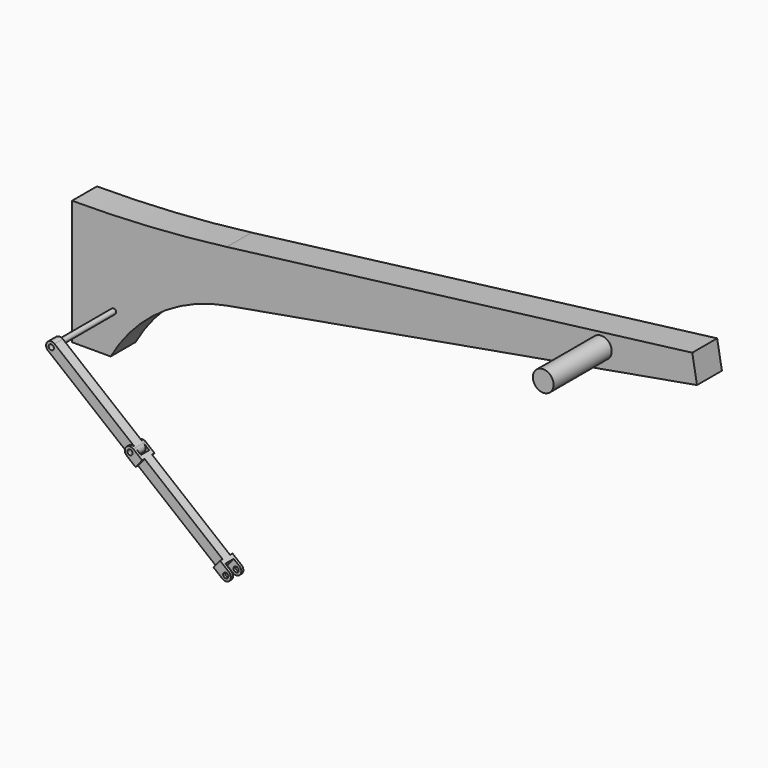
from build123d import *

# Parameters (mm, degrees)
F23_R     = 12.5
F25_DEPTH = 37.5
F24_R     = 12.5
F26_DEPTH = 25
F27_W     = 25
F27_H     = 25
F27_W_2   = 35
F27_W_3   = 482.723958417
F27_H_2   = 15
F28_DEPTH = 594.1776868073
F21_R     = 50
F30_DEPTH = 350
F29_R     = 12.5
F31_R     = 50
F32_DEPTH = 150


# Not quite as in the source:
# - a pattern or mirror of a feature is missing from the dataset's text; its kind, count and spacing are read off the source's solid


with BuildPart() as f25:
    # F23 (on Front) → F25 (new body, symmetric)
    with BuildSketch(Plane.XZ):
        with BuildLine():
            Line((-852.3729289945, 617.7499249904), (-391.0874269249, 245.5438309217))
            ThreePointArc((-391.0874269249, 245.5438309217), (-355.9322933967, 249.3010355502), (-359.6894980253, 284.4561690783))
            Line((-359.6894980253, 284.4561690783), (-820.9750000949, 656.6622631471))
            ThreePointArc((-820.9750000949, 656.6622631471), (-856.130133623, 652.9050585185), (-852.3729289945, 617.7499249904))
        make_face()
        with Locations((-375.3884624751, 265)):
            Circle(F23_R, mode=Mode.SUBTRACT)
        with Locations((-836.6739645447, 637.2060940687)):
            Circle(F23_R, mode=Mode.SUBTRACT)
    extrude(amount=F25_DEPTH, both=True)

    # F27 (on face) → F28 (cut, through all)
    with BuildSketch(Plane(origin=(-2.8214259663, 0, -3.4966727148), x_dir=(0.7782467631, 0, -0.627958578), z_dir=(0.627958578, 0, 0.7782467631))):
        with Locations((-446.0538790064, -12.5)):
            Rectangle(F27_W, F27_H)
        with Locations((-476.0538790064, -12.5)):
            Rectangle(F27_W_2, F27_H)
        with Locations((-754.9158582149, -30)):
            Rectangle(F27_W_3, F27_H_2)
        Polygon((-1051.2778374234, 0), (-1051.2778374234, -25), (-1026.2778374234, -25), (-1016.2778374234, -25), (-1016.2778374234, 0), align=None)
        with Locations((-1063.7778374234, -12.5)):
            Rectangle(F27_W, F27_H)
    f28 = extrude(amount=-F28_DEPTH, mode=Mode.SUBTRACT)

    # F28_copies: F28 across plane
    add(f28.mirror(Plane.ZX), mode=Mode.SUBTRACT)


with BuildPart() as f26:
    # F24 (on Front) → F26 (new body, symmetric)
    with BuildSketch(Plane.XZ):
        with BuildLine():
            Line((-1241.4963105611, 931.7292139859), (-852.3729289945, 617.7499249904))
            ThreePointArc((-852.3729289945, 617.7499249904), (-817.2177954663, 621.507129619), (-820.9750000949, 656.6622631471))
            Line((-820.9750000949, 656.6622631471), (-1210.0983816616, 970.6415521426))
            ThreePointArc((-1210.0983816616, 970.6415521426), (-1245.2535151897, 966.884347514), (-1241.4963105611, 931.7292139859))
        make_face()
        with Locations((-836.6739645447, 637.2060940687)):
            Circle(F24_R, mode=Mode.SUBTRACT)
        with Locations((-1225.7973461113, 951.1853830643)):
            Circle(F24_R, mode=Mode.SUBTRACT)
    extrude(amount=F26_DEPTH, both=True)


with BuildPart() as f30:
    # F21 (on Front) → F30 (new body)
    with BuildSketch(Plane.XZ):
        with Locations((1124.2026538887, 1562.1690044389)):
            Circle(F21_R)
    extrude(amount=-F30_DEPTH)



with BuildPart() as f30b:
    # F29 (on Front) → F30, piece 2 (new body)
    with BuildSketch(Plane.XZ):
        with Locations((-1225.7973461113, 951.1853830643)):
            Circle(F29_R)
    extrude(amount=-F30_DEPTH)


with BuildPart() as f30_1:
    add(f30.part)

    add(f30b.part)  # F32 merges F30b
    # F31 (on face) → F32 (join)
    with BuildSketch(Plane(origin=(0, 350, 0), x_dir=(-1, 0, 0), z_dir=(0, 1, 0))):
        with BuildLine():
            Line((1239.6273612976, 754.9997501798), (1425.7973461113, 754.9997501798))
            Line((1425.7973461113, 754.9997501798), (1425.7973461113, 1354.9997501798))
            ThreePointArc((1425.7973461113, 1354.9997501798), (1052.4711090827, 1366.6253864025), (680.5915903955, 1401.4572432645))
            Line((680.5915903955, 1401.4572432645), (-1562.0499747349, 1682.1690044389))
            Line((-1562.0499747349, 1682.1690044389), (-1584.972482227, 1552.1690044389))
            Line((-1584.972482227, 1552.1690044389), (680.085349701, 1152.7781958049))
            ThreePointArc((680.085349701, 1152.7781958049), (1004.6944340347, 1016.9612408233), (1239.6273612976, 754.9997501798))
        make_face()
        with Locations((-1124.2026538887, 1562.1690044389)):
            Circle(F31_R, mode=Mode.SUBTRACT)
        with Locations((-1124.2026538887, 1562.1690044389)):
            Circle(F31_R)
    extrude(amount=F32_DEPTH)


solid = Compound([f25.part, f26.part, f30_1.part])
